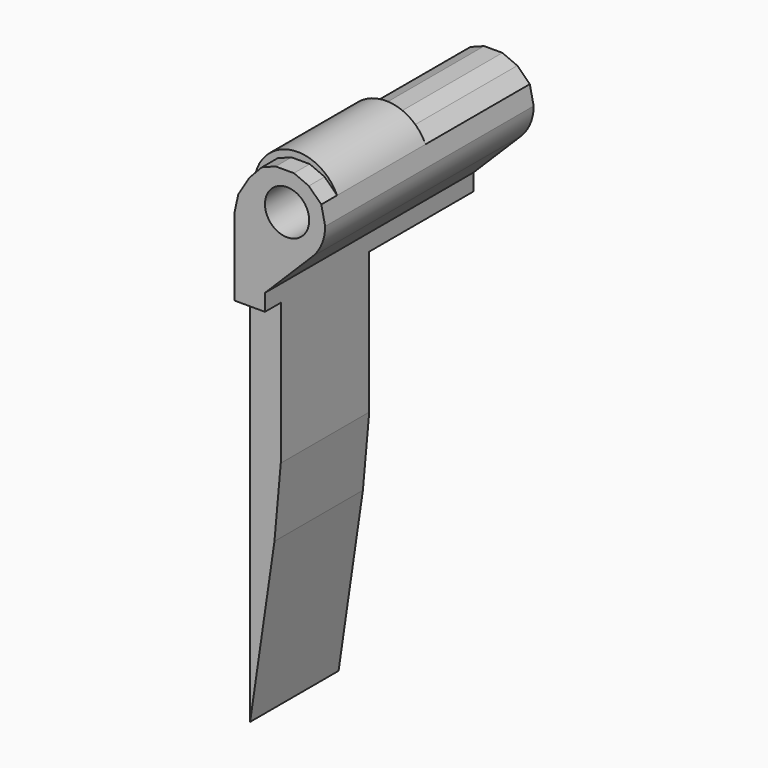
from build123d import *

# Parameters (mm, degrees)
F1_DEPTH = 8.25
F2_DEPTH = 7


# Not quite as in the source:
# - a feature names something its author has since deleted; it is built from what else it names


with BuildPart() as f1:
    # F0 (on Front) → F1 (new body, symmetric)
    with BuildSketch(Plane.XZ):
        with BuildLine():
            Line((-1.2599999983, 0.001106019), (-0.2481810163, 0.001106019))
            Line((-0.2481810241, 0.001106019), (-0.4941885147, 1.1379972147))
            Line((-0.4941885147, 1.1379972147), (-1.2832667135, 1.9140606746))
            Line((-1.2832667135, 1.9140606746), (-2.2277169394, 2.3196199825))
            Line((-2.2277169394, 2.3196199825), (-3.3833966788, 2.3196199825))
            Line((-3.3833966788, 2.3196199825), (-4.2535923825, 1.9888198258))
            Line((-4.2535923825, 1.9888198258), (-5.0546050044, 1.1417629963))
            Line((-5.0546050044, 1.1417629963), (-5.7481810085, 0.001106019))
            Line((-5.7481810085, 0.001106019), (-4.0599999983, 0.001106019))
            ThreePointArc((-4.0599999983, 0.001106019), (-2.6599999983, 1.401106019), (-1.2599999983, 0.001106019))
        make_face()
        with BuildLine():
            ThreePointArc((-1.0547499373, -1.9445495701), (-0.4578133732, -1.0519999951), (-0.2481810085, 0.001106019))
            Line((-0.2481810163, 0.001106019), (-1.2599999983, 0.001106019))
            ThreePointArc((-1.2599999983, 0.001106019), (-2.6599999983, -1.398893981), (-4.0599999983, 0.001106019))
            Line((-4.0599999983, 0.001106019), (-5.7481810085, 0.001106019))
            ThreePointArc((-5.7481810085, 0.001106019), (-4.0512870227, -2.5392616163), (-1.0547499373, -1.9445495701))
        make_face()
        with BuildLine():
            Line((-4.0599999966, -4.9463636499), (-1.0547499373, -1.9445495701))
            ThreePointArc((-1.0547499373, -1.9445495701), (-4.0512870227, -2.5392616163), (-5.7481810085, 0.001106019))
            Line((-5.7481810085, 0.001106019), (-5.9999999983, -1.1473703696))
            Line((-5.9999999983, -1.1473703696), (-5.9999999983, -4.8066070303))
            Line((-5.9999999983, -4.8066070303), (-5.9999999983, -6.0053556226))
            Line((-5.9999999983, -6.0053556226), (-5.1202041279, -6.0053556226))
            Line((-5.1202041279, -6.0053556226), (-4.0599999966, -4.9463636499))
        make_face()
        Polygon((-4.0599999966, -6.0053556226), (-4.0599999966, -4.9463636499), (-5.1202041279, -6.0053556226), align=None)
    extrude(amount=F1_DEPTH, both=True)

    # F0 (on Front) → F2 (join)
    with BuildSketch(Plane.XZ):
        with BuildLine():
            Line((-1.2832667135, 1.9140606746), (-0.4941885147, 1.1379972147))
            ThreePointArc((-0.4941885147, 1.1379972147), (-3.5797825225, 2.6889005943), (-5.7481810085, 0.001106019))
            Line((-5.7481810085, 0.001106019), (-5.0546050044, 1.1417629963))
            Line((-5.0546050044, 1.1417629963), (-4.2535923825, 1.9888198258))
            Line((-4.2535923825, 1.9888198258), (-3.3833966788, 2.3196199825))
            Line((-3.3833966788, 2.3196199825), (-2.2277169394, 2.3196199825))
            Line((-2.2277169394, 2.3196199825), (-1.2832667135, 1.9140606746))
        make_face()
        Polygon((-5.9999999983, -1.1473703696), (-5.7481810085, 0.001106019), (-6, 0.001106019), align=None)
        Polygon((-4.0599999966, -14.9466558945), (-4.0599999966, -8.645166643), (-5.9999999983, -8.645166643), (-5.9999999983, -30), (-4.4599999966, -19.4339305162), align=None)
        Polygon((-4.0599999966, -6.0053556226), (-5.1202041279, -6.0053556226), (-6, -6.8841456016), (-5.9999999983, -8.645166643), (-4.0599999966, -8.645166643), align=None)
        Polygon((-6, -6.8841456016), (-5.1202041279, -6.0053556226), (-5.9999999983, -6.0053556226), align=None)
    extrude(amount=F2_DEPTH)


solid = f1.part
